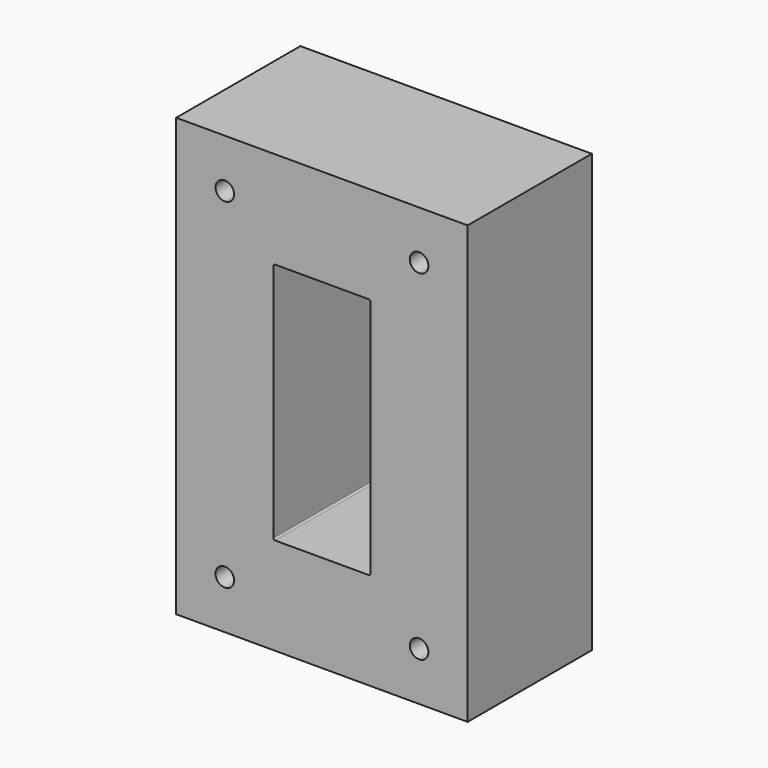
from build123d import *

# Parameters (mm, degrees)
F1_W     = 137.16
F1_H     = 205.74
F2_DEPTH = 73.025
F3_R     = 4.365625
F4_DEPTH = 73.025
F5_W     = 45.72
F5_H     = 114.3
F6_DEPTH = 73.025
F7_R     = 0.79375


# Not quite as in the source:
# - a variable given as a bare number and used for a length is read in inches; the dataset says mm whatever the document's units were


with BuildPart() as f2:
    # F1 (on Front) → F2 (new body)
    with BuildSketch(Plane.XZ):
        Rectangle(F1_W, F1_H)
    extrude(amount=-F2_DEPTH)

    # F3 (on face) → F4 (cut)
    with BuildSketch(Plane.XZ):
        with Locations((-45.72, 80.01)):
            Circle(F3_R)
        with Locations((45.72, 80.01)):
            Circle(F3_R)
        with Locations((-45.72, -80.01)):
            Circle(F3_R)
        with Locations((45.72, -80.01)):
            Circle(F3_R)
    extrude(amount=-F4_DEPTH, mode=Mode.SUBTRACT)

    # F5 (on face) → F6 (cut)
    with BuildSketch(Plane.XZ):
        Rectangle(F5_W, F5_H)
    extrude(amount=-F6_DEPTH, mode=Mode.SUBTRACT)

    # F7
    f7_edges = [f2.edges().sort_by_distance(p)[0] for p in [
        (-22.86, 36.5125, 57.15),
        (22.86, 36.5125, 57.15),
        (22.86, 36.5125, -57.15),
        (-22.86, 36.5125, -57.15),
    ]]
    fillet(f7_edges, radius=F7_R)


solid = f2.part
